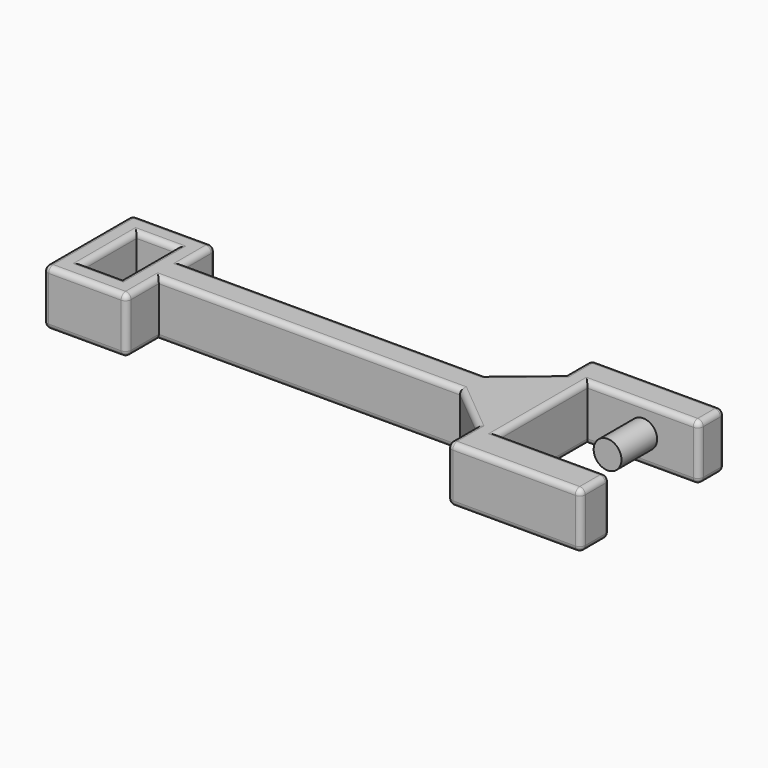
from build123d import *

# Parameters (mm, degrees)
F0_W     = 8.89
F0_H     = 15.24
F1_DEPTH = 12.7
F2_R     = 3.175
F5_DEPTH = 10.16
F6_R     = 1.27


# Not quite as in the source:
# - the program builds the solid bodies; features that only make, move or delete a surface that nothing else refers to are left out


with BuildPart() as f1:
    # F0 (on Top) → F1 (new body)
    with BuildSketch(Plane.XY):
        Polygon((-12.7, 12.7), (12.7, 12.7), (12.7, 20.1094653457), (-17.78, 20.1094653457), (-17.78, 12.7), (-28.8291541207, 3.5404531619), (-97.5522994995, 3.5404531619), (-97.5522994995, 12.7), (-116.6022994995, 12.7), (-116.6022994995, -12.7), (-97.5522994995, -12.7), (-97.5522994995, -3.5404531619), (-28.8291541207, -3.5404531619), (-17.78, -12.7), (-17.78, -20.9651887417), (12.7, -20.9651887417), (12.7, -12.7), (-12.7, -12.7), align=None)
        with Locations((-107.0772994995, 0)):
            Rectangle(F0_W, F0_H, mode=Mode.SUBTRACT)
    extrude(amount=F1_DEPTH)

    # F2 (on face) → F5 (join)
    with BuildSketch(Plane.XZ.offset(-12.7)):
        with Locations((0, 6.35)):
            Circle(F2_R)
    extrude(amount=F5_DEPTH)

    # F6
    f6_edges = [f1.edges().sort_by_distance(p)[0] for p in [
        (-63.190727, -3.540453, 12.7),
        (-63.190727, 3.540453, 12.7),
        (-63.190727, -3.540453, 0),
        (-107.077299, -12.7, 12.7),
        (-97.552299, -8.120227, 12.7),
        (-97.552299, -12.7, 6.35),
        (-97.552299, -8.120227, 0),
        (-107.077299, -12.7, 0),
        (-116.602299, -12.7, 6.35),
        (-116.602299, 0, 12.7),
        (-107.077299, 12.7, 12.7),
        (-97.552299, 8.120227, 12.7),
        (-102.632299, 0, 12.7),
        (-107.077299, 7.62, 12.7),
        (-111.522299, 0, 12.7),
        (-107.077299, -7.62, 12.7),
        (-116.602299, 12.7, 6.35),
        (-116.602299, 0, 0),
        (-111.522299, 0, 0),
        (-107.077299, 7.62, 0),
        (-102.632299, 0, 0),
        (-107.077299, -7.62, 0),
        (-107.077299, 12.7, 0),
        (-97.552299, 12.7, 6.35),
        (-97.552299, 8.120227, 0),
        (-63.190727, 3.540453, 0),
        (-17.78, 20.109465, 6.35),
        (-23.304577, 8.120227, 12.7),
        (-23.304577, 8.120227, 0),
        (-17.78, 16.404733, 0),
        (-17.78, 16.404733, 12.7),
        (-2.54, 20.109465, 12.7),
        (-2.54, 20.109465, 0),
        (0, 12.7, 0),
        (12.7, 16.404733, 0),
        (12.7, 20.109465, 6.35),
        (12.7, -12.7, 6.35),
        (0, -12.7, 0),
        (12.7, -16.832594, 0),
        (-2.54, -20.965189, 0),
        (-17.78, -16.832594, 0),
        (-12.7, 0, 0),
        (-23.304577, -8.120227, 0),
        (-23.304577, -8.120227, 12.7),
        (-12.7, 0, 12.7),
        (0, 12.7, 12.7),
        (12.7, 16.404733, 12.7),
        (12.7, 12.7, 6.35),
        (-17.78, -16.832594, 12.7),
        (-17.78, -20.965189, 6.35),
        (-2.54, -20.965189, 12.7),
        (0, -12.7, 12.7),
        (12.7, -16.832594, 12.7),
        (12.7, -20.965189, 6.35),
    ]]
    fillet(f6_edges, radius=F6_R)


solid = f1.part
